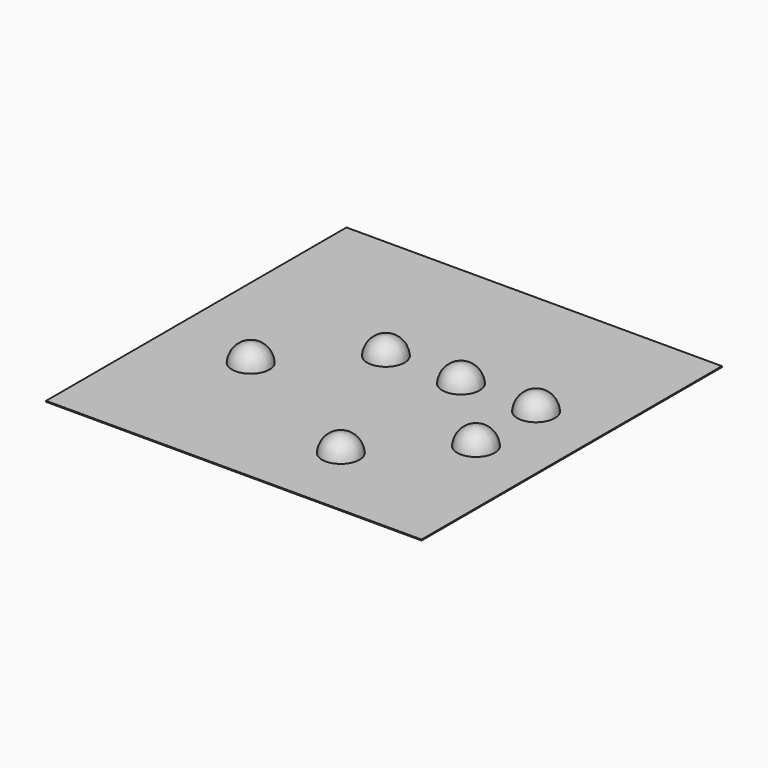
from build123d import *

# Parameters (mm, degrees)
F0_W     = 200
F0_H     = 200
F2_DEPTH = 0.5
F1_R     = 10
F3_DEPTH = 10


# Not quite as in the source:
# - a fillet or chamfer that OpenCascade refuses, or shapes differently, is made with other operations: its cross-section is extruded or revolved along the edge and cut away or added


with BuildPart() as f2:
    # F0 (on Top) → F2 (new body)
    with BuildSketch(Plane.XY):
        Rectangle(F0_W, F0_H)
    extrude(amount=F2_DEPTH)

    # F1 (on face) → F3 (join)
    with BuildSketch(Plane.XY):
        with Locations((-55, -20)):
            Circle(F1_R)
        with Locations((-15, 20)):
            Circle(F1_R)
        with Locations((25, -60)):
            Circle(F1_R)
        with Locations((25, 20)):
            Circle(F1_R)
        with Locations((65, -20)):
            Circle(F1_R)
        with Locations((65, 20)):
            Circle(F1_R)
    extrude(amount=F3_DEPTH)

    # F4: fillet of radius 10 on 6 edges, made by hand

    # F4_s1 → F4_t2 (revolve, cut)
    with BuildSketch(Plane.XZ.offset(20)):
        with BuildLine():
            ThreePointArc((-45, 0.5), (-48.0954678017, 7.2456883731), (-54.9874921777, 10))
            Line((-54.9874921777, 10), (-45, 10))
            Line((-45, 10), (-45, 0.5))
        make_face()
    revolve(axis=Axis((-55, -20, 10), (0, 0, 1)), mode=Mode.SUBTRACT)

    # F4_s3 → F4_t4 (revolve, cut)
    with BuildSketch(Plane.XZ.offset(-20)):
        with BuildLine():
            ThreePointArc((-5, 0.5), (-8.0954678017, 7.2456883731), (-14.9874921777, 10))
            Line((-14.9874921777, 10), (-5, 10))
            Line((-5, 10), (-5, 0.5))
        make_face()
    revolve(axis=Axis((-15, 20, 10), (0, 0, 1)), mode=Mode.SUBTRACT)

    # F4_s5 → F4_t6 (revolve, cut)
    with BuildSketch(Plane.XZ.offset(-20)):
        with BuildLine():
            ThreePointArc((35, 0.5), (31.9045321983, 7.2456883731), (25.0125078223, 10))
            Line((25.0125078223, 10), (35, 10))
            Line((35, 10), (35, 0.5))
        make_face()
    revolve(axis=Axis((25, 20, 10), (0, 0, 1)), mode=Mode.SUBTRACT)

    # F4_s7 → F4_t8 (revolve, cut)
    with BuildSketch(Plane.XZ.offset(-20)):
        with BuildLine():
            ThreePointArc((75, 0.5), (71.9045321983, 7.2456883731), (65.0125078223, 10))
            Line((65.0125078223, 10), (75, 10))
            Line((75, 10), (75, 0.5))
        make_face()
    revolve(axis=Axis((65, 20, 10), (0, 0, 1)), mode=Mode.SUBTRACT)

    # F4_s9 → F4_t10 (revolve, cut)
    with BuildSketch(Plane.XZ.offset(20)):
        with BuildLine():
            ThreePointArc((75, 0.5), (71.9045321983, 7.2456883731), (65.0125078223, 10))
            Line((65.0125078223, 10), (75, 10))
            Line((75, 10), (75, 0.5))
        make_face()
    revolve(axis=Axis((65, -20, 10), (0, 0, 1)), mode=Mode.SUBTRACT)

    # F4_s11 → F4_t12 (revolve, cut)
    with BuildSketch(Plane.XZ.offset(60)):
        with BuildLine():
            ThreePointArc((35, 0.5), (31.9045321983, 7.2456883731), (25.0125078223, 10))
            Line((25.0125078223, 10), (35, 10))
            Line((35, 10), (35, 0.5))
        make_face()
    revolve(axis=Axis((25, -60, 10), (0, 0, 1)), mode=Mode.SUBTRACT)


solid = f2.part
